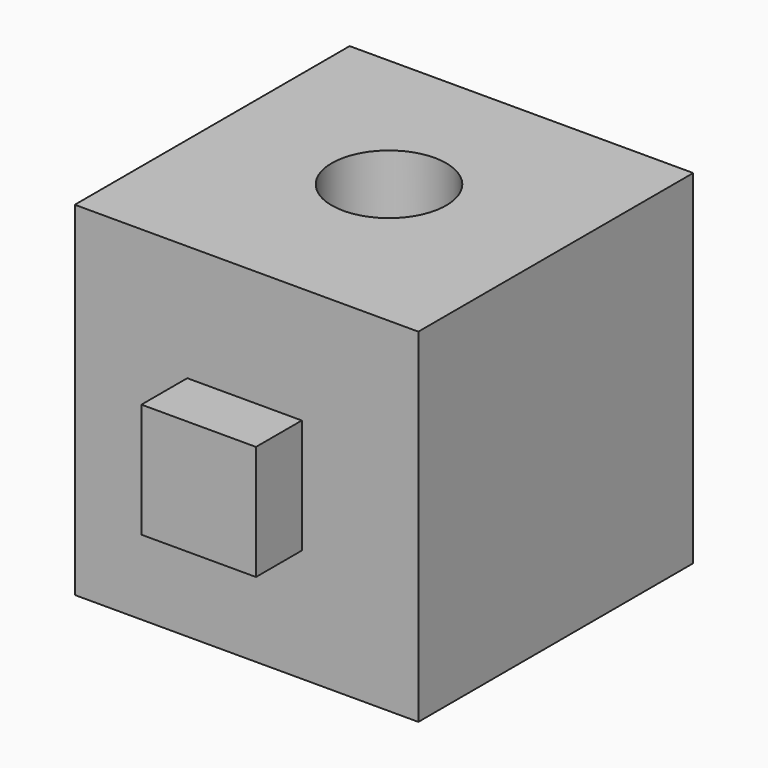
from build123d import *

# Parameters (mm, degrees)
F0_W     = 76.2
F0_H     = 76.2
F1_DEPTH = 76.2
F3_D     = 25.4
F4_W     = 25.4
F4_H     = 25.4
F5_DEPTH = 12.7


# Not quite as in the source:
# - the program builds the solid bodies; features that only make, move or delete a surface that nothing else refers to are left out


with BuildPart() as f1:
    # F0 (on Front) → F1 (new body)
    with BuildSketch(Plane.XZ):
        with Locations((38.1, 38.1)):
            Rectangle(F0_W, F0_H)
    extrude(amount=F1_DEPTH)

    # F3 (through all)
    with Locations(Plane.XY.offset(76.2)):
        with Locations((37.7037897706, -36.2189039588)):
            Hole(F3_D / 2)

    # F4 (on face) → F5 (join)
    with BuildSketch(Plane.XZ.offset(76.2)):
        with Locations((37.6457564205, 37.7473003834)):
            Rectangle(F4_W, F4_H)
    extrude(amount=F5_DEPTH)


solid = f1.part
